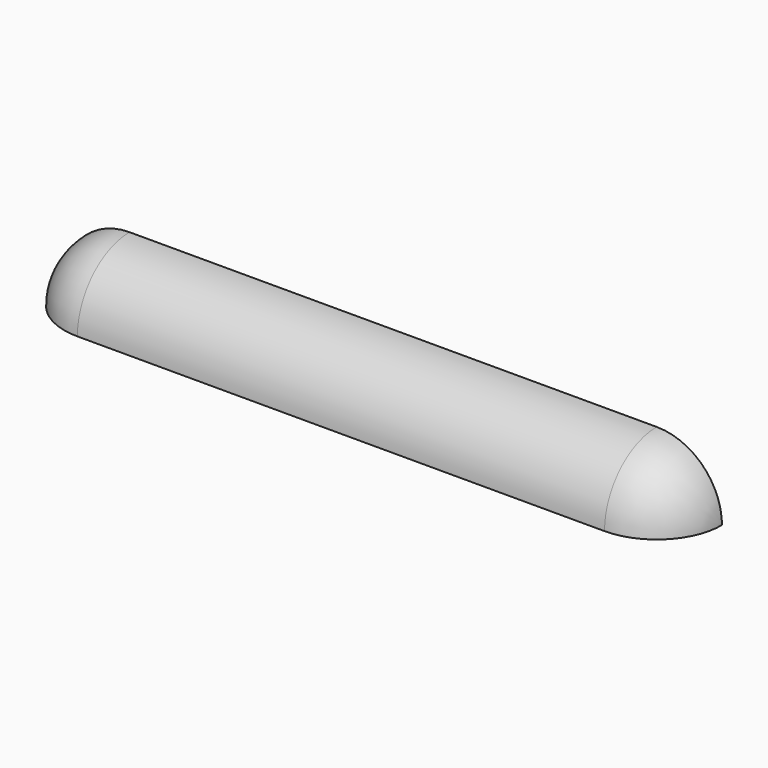
from build123d import *

# Parameters (mm, degrees)
F1_DEPTH = 50.4
F2_R     = 9.99999


# Not quite as in the source:
# - a fillet or chamfer is up to 0.001 mm smaller than in the source, because OpenCascade refuses the exact size


with BuildPart() as f1:
    # F0 (on Right) → F1 (new body, symmetric)
    with BuildSketch(Plane.YZ):
        with BuildLine():
            Line((-5, -5), (5, -5))
            Line((5, -5), (5, 5))
            ThreePointArc((5, 5), (-2.0710678119, 2.0710678119), (-5, -5))
        make_face()
    extrude(amount=F1_DEPTH, both=True)

    # F2 (radius 10 in the source; OpenCascade refuses exactly that, so slightly less here)
    f2_edges = [f1.edges().sort_by_distance(p)[0] for p in [
        (50.4, -2.071068, 2.071068),
        (-50.4, -2.071068, 2.071068),
    ]]
    fillet(f2_edges, radius=F2_R)


solid = f1.part
